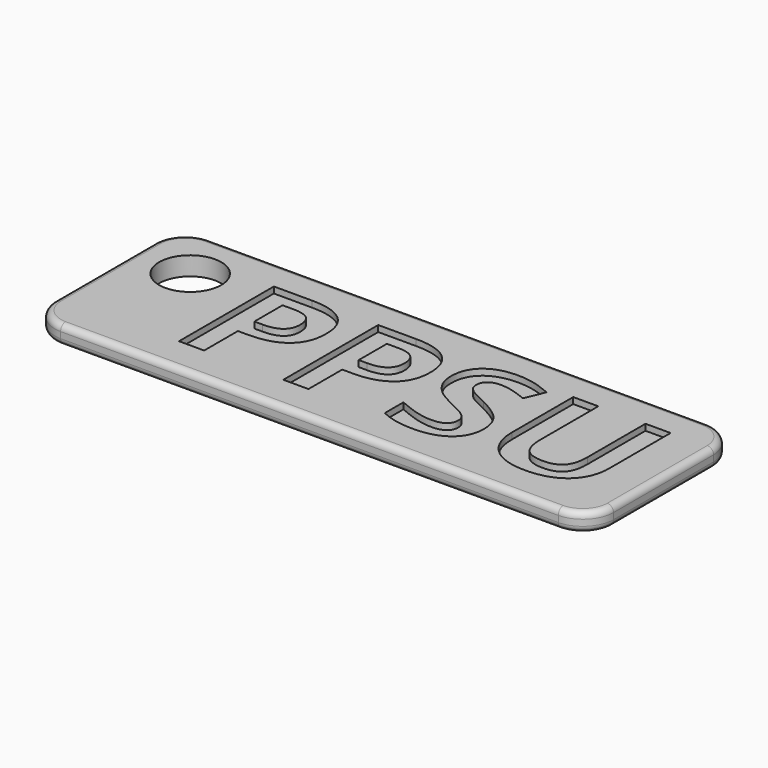
from build123d import *

# Parameters (mm, degrees)
F0_W         = 90
F0_H         = 30
F1_DEPTH     = 3
F2_R         = 1
F3_T1_DEPTH  = 3
F3_T4_ANGLE  = 90
F3_T6_ANGLE  = 90
F3_T8_ANGLE  = 90
F3_T10_ANGLE = 90
F3_T12_ANGLE = 90
F3_T14_ANGLE = 90
F3_T16_ANGLE = 90
F3_T18_ANGLE = 90
F4_R         = 5
F5_DEPTH     = 3
F6_TEXT_SIZE = 26.7453294002
F7_DEPTH     = 1


# Not quite as in the source:
# - a fillet or chamfer that OpenCascade refuses, or shapes differently, is made with other operations: its cross-section is extruded or revolved along the edge and cut away or added
# - Text() gives the source's letters only with a copy of the font that has no kerning and outlines rounded to 1/6400 em; it was checked with that copy


with BuildPart() as f1:
    # F0 (on Top) → F1 (new body)
    with BuildSketch(Plane.XY):
        Rectangle(F0_W, F0_H)
    extrude(amount=F1_DEPTH)

    # F2
    f2_edges = [f1.edges().sort_by_distance(p)[0] for p in [
        (0, 15, 3),
        (-45, 0, 3),
        (0, -15, 3),
        (45, 0, 3),
        (0, 15, 0),
        (-45, 0, 0),
        (0, -15, 0),
        (45, 0, 0),
    ]]
    fillet(f2_edges, radius=F2_R)

    # F3: fillet of radius 5 on 4 edges, made by hand

    # F3_s2 → F3_t1 (cut)
    with BuildSketch(Plane.XY):
        with BuildLine():
            ThreePointArc((45.0004, -9.9990343146), (43.5355339059, -13.5355339059), (39.9990343146, -15.0004))
            Line((39.9990343146, -15.0004), (39.9990343146, -15.5005365685))
            ThreePointArc((39.9990343146, -15.5005365685), (42.4995171573, -15.5001365685), (45, -15.5001365685))
            Line((45, -15.5001365685), (45.5001365685, -15))
            ThreePointArc((45.5001365685, -15), (45.5001365685, -12.4995171573), (45.5005365685, -9.9990343146))
            Line((45.5005365685, -9.9990343146), (45.0004, -9.9990343146))
        make_face()
        with BuildLine():
            ThreePointArc((39.9990343146, 15.0004), (43.5355339059, 13.5355339059), (45.0004, 9.9990343146))
            Line((45.0004, 9.9990343146), (45.5005365685, 9.9990343146))
            ThreePointArc((45.5005365685, 9.9990343146), (45.5001365685, 12.4995171573), (45.5001365685, 15))
            Line((45.5001365685, 15), (45, 15.5001365685))
            ThreePointArc((45, 15.5001365685), (42.4995171573, 15.5001365685), (39.9990343146, 15.5005365685))
            Line((39.9990343146, 15.5005365685), (39.9990343146, 15.0004))
        make_face()
        with BuildLine():
            ThreePointArc((-39.9990343146, 15.0004), (-43.5355339059, 13.5355339059), (-45.0004, 9.9990343146))
            Line((-45.0004, 9.9990343146), (-45.5005365685, 9.9990343146))
            ThreePointArc((-45.5005365685, 9.9990343146), (-45.5001365685, 12.4995171573), (-45.5001365685, 15))
            Line((-45.5001365685, 15), (-45, 15.5001365685))
            ThreePointArc((-45, 15.5001365685), (-42.4995171573, 15.5001365685), (-39.9990343146, 15.5005365685))
            Line((-39.9990343146, 15.5005365685), (-39.9990343146, 15.0004))
        make_face()
        with BuildLine():
            ThreePointArc((-45.0004, -9.9990343146), (-43.5355339059, -13.5355339059), (-39.9990343146, -15.0004))
            Line((-39.9990343146, -15.0004), (-39.9990343146, -15.5005365685))
            ThreePointArc((-39.9990343146, -15.5005365685), (-42.4995171573, -15.5001365685), (-45, -15.5001365685))
            Line((-45, -15.5001365685), (-45.5001365685, -15))
            ThreePointArc((-45.5001365685, -15), (-45.5001365685, -12.4995171573), (-45.5005365685, -9.9990343146))
            Line((-45.5005365685, -9.9990343146), (-45.0004, -9.9990343146))
        make_face()
    extrude(amount=F3_T1_DEPTH, mode=Mode.SUBTRACT)

    # F3_s3 → F3_t4 (revolve, cut)
    with BuildSketch(Plane.YZ.offset(-39.9990343146)):
        with BuildLine():
            ThreePointArc((-14.0004, 0), (-14.7075067812, 0.2928932188), (-15.0004, 1))
            Line((-15.0004, 1), (-15.0004, 0))
            Line((-15.0004, 0), (-14.0004, 0))
        make_face()
    revolve(axis=Axis((-39.9990343146, -9.9990343146, 0), (0, 0, -1)), revolution_arc=F3_T4_ANGLE, mode=Mode.SUBTRACT)

    # F3_s5 → F3_t6 (revolve, cut)
    with BuildSketch(Plane.XZ.offset(9.9990343146)):
        with BuildLine():
            ThreePointArc((-44.0004, 3), (-44.7075067812, 2.7071067812), (-45.0004, 2))
            Line((-45.0004, 2), (-45.0004, 3))
            Line((-45.0004, 3), (-44.0004, 3))
        make_face()
    revolve(axis=Axis((-39.9990343146, -9.9990343146, 3), (0, 0, 1)), revolution_arc=F3_T6_ANGLE, mode=Mode.SUBTRACT)

    # F3_s7 → F3_t8 (revolve, cut)
    with BuildSketch(Plane.XZ.offset(-9.9990343146)):
        with BuildLine():
            ThreePointArc((-44.0004, 0), (-44.7075067812, 0.2928932188), (-45.0004, 1))
            Line((-45.0004, 1), (-45.0004, 0))
            Line((-45.0004, 0), (-44.0004, 0))
        make_face()
    revolve(axis=Axis((-39.9990343146, 9.9990343146, 0), (0, 0, -1)), revolution_arc=F3_T8_ANGLE, mode=Mode.SUBTRACT)

    # F3_s9 → F3_t10 (revolve, cut)
    with BuildSketch(Plane.YZ.offset(-39.9990343146)):
        with BuildLine():
            ThreePointArc((14.0004, 3), (14.7075067812, 2.7071067812), (15.0004, 2))
            Line((15.0004, 2), (15.0004, 3))
            Line((15.0004, 3), (14.0004, 3))
        make_face()
    revolve(axis=Axis((-39.9990343146, 9.9990343146, 3), (0, 0, 1)), revolution_arc=F3_T10_ANGLE, mode=Mode.SUBTRACT)

    # F3_s11 → F3_t12 (revolve, cut)
    with BuildSketch(Plane.YZ.offset(39.9990343146)):
        with BuildLine():
            ThreePointArc((14.0004, 0), (14.7075067812, 0.2928932188), (15.0004, 1))
            Line((15.0004, 1), (15.0004, 0))
            Line((15.0004, 0), (14.0004, 0))
        make_face()
    revolve(axis=Axis((39.9990343146, 9.9990343146, 0), (0, 0, -1)), revolution_arc=F3_T12_ANGLE, mode=Mode.SUBTRACT)

    # F3_s13 → F3_t14 (revolve, cut)
    with BuildSketch(Plane.XZ.offset(-9.9990343146)):
        with BuildLine():
            ThreePointArc((44.0004, 3), (44.7075067812, 2.7071067812), (45.0004, 2))
            Line((45.0004, 2), (45.0004, 3))
            Line((45.0004, 3), (44.0004, 3))
        make_face()
    revolve(axis=Axis((39.9990343146, 9.9990343146, 3), (0, 0, 1)), revolution_arc=F3_T14_ANGLE, mode=Mode.SUBTRACT)

    # F3_s15 → F3_t16 (revolve, cut)
    with BuildSketch(Plane.XZ.offset(9.9990343146)):
        with BuildLine():
            ThreePointArc((44.0004, 0), (44.7075067812, 0.2928932188), (45.0004, 1))
            Line((45.0004, 1), (45.0004, 0))
            Line((45.0004, 0), (44.0004, 0))
        make_face()
    revolve(axis=Axis((39.9990343146, -9.9990343146, 0), (0, 0, -1)), revolution_arc=F3_T16_ANGLE, mode=Mode.SUBTRACT)

    # F3_s17 → F3_t18 (revolve, cut)
    with BuildSketch(Plane.YZ.offset(39.9990343146)):
        with BuildLine():
            ThreePointArc((-14.0004, 3), (-14.7075067812, 2.7071067812), (-15.0004, 2))
            Line((-15.0004, 2), (-15.0004, 3))
            Line((-15.0004, 3), (-14.0004, 3))
        make_face()
    revolve(axis=Axis((39.9990343146, -9.9990343146, 3), (0, 0, 1)), revolution_arc=F3_T18_ANGLE, mode=Mode.SUBTRACT)

    # F4 (on face) → F5 (cut)
    with BuildSketch(Plane.XY.offset(3)):
        with Locations((-36, 6)):
            Circle(F4_R)
    extrude(amount=-F5_DEPTH, mode=Mode.SUBTRACT)

    # F6 (on face) → F7 (cut)
    with BuildSketch(Plane.XY.offset(3)):
        with Locations((-28, -9.2566371681)):
            Text('PPSU', F6_TEXT_SIZE, font='Open Sans', font_style=FontStyle.BOLD, text_align=(TextAlign.LEFT, TextAlign.BOTTOM))
    extrude(amount=-F7_DEPTH, mode=Mode.SUBTRACT)


solid = f1.part
